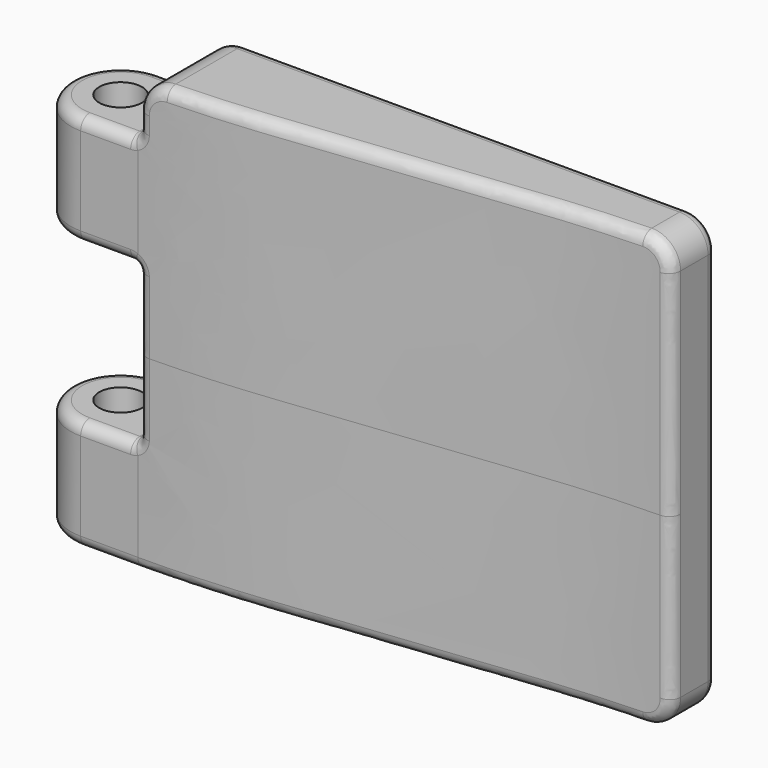
from build123d import *

# Parameters (mm, degrees)
F0_R          = 1.5
F1_DEPTH      = 13.3
F3_DEPTH      = 17
F3_DEPTH_BACK = 13.3
F4_DEPTH      = 5.525
F5_T1_DEPTH   = 7
F6_R          = 2
F7_R          = 0.8


# Not quite as in the source:
# - a fillet or chamfer that OpenCascade refuses, or shapes differently, is made with other operations: its cross-section is extruded or revolved along the edge and cut away or added


with BuildPart() as f1:
    # F0 (on Top) → F1 (new body, symmetric)
    with BuildSketch(Plane.XY):
        with BuildLine():
            ThreePointArc((-4, 0), (-7.5, -3.5), (-4, -7))
            Line((-4, -7), (0, -7))
            Line((0, -7), (0, 0))
            Line((0, 0), (-4, 0))
        make_face()
        with Locations((-4, -3.5)):
            Circle(F0_R, mode=Mode.SUBTRACT)
    extrude(amount=F1_DEPTH, both=True)

    # F2 (on Top) → F3 (join, two sides)
    with BuildSketch(Plane.XY) as f3_sk:
        with BuildLine():
            Line((35, 0), (0, 0))
            Line((0, 0), (0, -7))
            add(Edge.make_bspline(
                [(35, -4), (30, -4), (22.19484358, -5.034570371), (12.80515642, -5.965429629), (5, -7), (0, -7)],
                knots=[0, 0, 0, 0, 0.3529358035, 0.6470641965, 1, 1, 1, 1], degree=3))
            Line((35, -4), (35, 0))
        make_face()
    extrude(amount=F3_DEPTH)
    extrude(f3_sk.sketch, amount=-F3_DEPTH_BACK)

    # F0 (on Top) → F4 (cut, symmetric)
    with BuildSketch(Plane.XY):
        with BuildLine():
            ThreePointArc((-4, 0), (-7.5, -3.5), (-4, -7))
            Line((-4, -7), (0, -7))
            Line((0, -7), (0, 0))
            Line((0, 0), (-4, 0))
        make_face()
        with Locations((-4, -3.5)):
            Circle(F0_R, mode=Mode.SUBTRACT)
    extrude(amount=F4_DEPTH, both=True, mode=Mode.SUBTRACT)

    # F5: fillet of radius 0.5 on 3 edges, made by hand

    # F5_s2 → F5_t1 (join)
    with BuildSketch(Plane.XZ):
        with BuildLine():
            ThreePointArc((0, 13.8), (-0.1464466094, 13.4464466094), (-0.5, 13.3))
            Line((-0.5, 13.3), (0, 13.3))
            Line((0, 13.3), (0, 13.8))
        make_face()
        with BuildLine():
            ThreePointArc((-0.5, 5.525), (-0.1464466094, 5.3785533906), (0, 5.025))
            Line((0, 5.025), (0, 5.525))
            Line((0, 5.525), (-0.5, 5.525))
        make_face()
        with BuildLine():
            ThreePointArc((-0.5, -5.525), (-0.1464466094, -5.3785533906), (0, -5.025))
            Line((0, -5.025), (0, -5.525))
            Line((0, -5.525), (-0.5, -5.525))
        make_face()
    extrude(amount=F5_T1_DEPTH)

    # F6
    f6_edges = [f1.edges().sort_by_distance(p)[0] for p in [
        (0, -3.5, 17),
        (35, -2, 17),
        (35, -2, -13.3),
    ]]
    fillet(f6_edges, radius=F6_R)

    # F7
    f7_edges = [f1.edges().sort_by_distance(p)[0] for p in [
        (35, -4, -5.65),
        (34.41412, -4.002571, -12.714307),
        (17.5, -5.5, 0),
        (16.505684, -5.607828, -13.3),
        (0, -7, -2.5125),
        (0, -7, -9.1625),
        (14.5, 0, -13.3),
        (34.414214, 0, -12.714214),
        (-4, 0, -9.4125),
        (35, 0, 1.85),
        (-2.25, 0, -5.525),
        (34.414214, 0, 16.414214),
        (-0.146447, 0, -5.378553),
        (17.5, 0, 17),
        (0, 0, 0),
        (0.585786, 0, 16.414214),
        (-0.146447, 0, 5.378553),
        (0, 0, 14.4),
        (-2.25, 0, 5.525),
        (-0.146447, 0, 13.446447),
        (-4, 0, 9.4125),
        (-2.25, 0, 13.3),
    ]]
    fillet(f7_edges, radius=F7_R)


solid = f1.part
